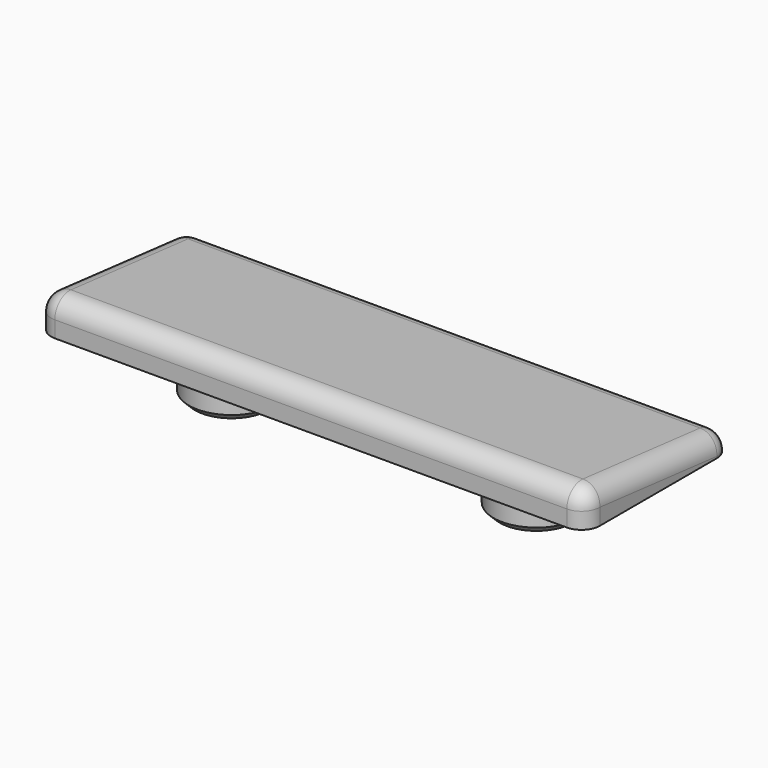
from build123d import *

# Parameters (mm, degrees)
F1_DEPTH     = 90
F3_R         = 7
F4_DEPTH     = 9
F5_R         = 3.35
F6_DEPTH     = 6
F7_SIZE      = 1
F8_R         = 3
F9_T1_DEPTH  = 84
F9_T3_DEPTH  = 24.1197014907
F9_T8_DEPTH  = 3
F9_T14_DEPTH = 3
F9_T20_DEPTH = 3
F9_T26_DEPTH = 3


# Not quite as in the source:
# - a fillet or chamfer that OpenCascade refuses, or shapes differently, is made with other operations: its cross-section is extruded or revolved along the edge and cut away or added


with BuildPart() as f1:
    # F0 (on Right) → F1 (new body)
    with BuildSketch(Plane.YZ):
        Polygon((-15, 6), (-15, 0), (15, 0), (15, 3), align=None)
    extrude(amount=F1_DEPTH)

    # F3 (on face) → F4 (join)
    with BuildSketch(Plane(origin=(0, 0, 0), x_dir=(1, 0, 0), z_dir=(0, 0, -1))):
        with Locations((70, 0)):
            Circle(F3_R)
        with Locations((20, 0)):
            Circle(F3_R)
    extrude(amount=F4_DEPTH)

    # F5 (on face) → F6 (cut)
    with BuildSketch(Plane(origin=(0, 0, -9), x_dir=(1, 0, 0), z_dir=(0, 0, -1))):
        with Locations((70, 0)):
            Circle(F5_R)
        with Locations((20, 0)):
            Circle(F5_R)
    extrude(amount=-F6_DEPTH, mode=Mode.SUBTRACT)

    # F7
    f7_edges = [f1.edges().sort_by_distance(p)[0] for p in [
        (63, 0, -9),
        (13, 0, -9),
    ]]
    chamfer(f7_edges, length=F7_SIZE)

    # F8
    f8_edges = [f1.edges().sort_by_distance(p)[0] for p in [
        (90, 15, 1.5),
        (0, 15, 1.5),
        (0, -15, 3),
        (90, -15, 3),
    ]]
    fillet(f8_edges, radius=F8_R)

    # F9: fillet of radius 3 on 4 edges, made by hand

    # F9_s2 → F9_t1 (cut)
    with BuildSketch(Plane.YZ.offset(3)):
        with BuildLine():
            ThreePointArc((15, 0.2850373137), (14.2243576007, 2.2980532759), (12.2985111571, 3.2701488843))
            Line((12.2985111571, 3.2701488843), (15, 3))
            Line((15, 3), (15, 0.2850373137))
        make_face()
        with BuildLine():
            ThreePointArc((-15, 2.6850373137), (-14.0130159623, 4.9093949143), (-11.7014888429, 5.6701488843))
            Line((-11.7014888429, 5.6701488843), (-15, 6))
            Line((-15, 6), (-15, 2.6850373137))
        make_face()
    extrude(amount=F9_T1_DEPTH, mode=Mode.SUBTRACT)

    # F9_s4 → F9_t3 (cut)
    with BuildSketch(Plane(origin=(0, 11.8529666026, -1.1852966603), x_dir=(1, 0, 0), z_dir=(0, -0.9950371902, 0.099503719))):
        with BuildLine():
            ThreePointArc((0, 1.4776673559), (0.8786796564, 3.5989876995), (3, 4.4776673559))
            Line((3, 4.4776673559), (0, 4.4776673559))
            Line((0, 4.4776673559), (0, 1.4776673559))
        make_face()
        with BuildLine():
            ThreePointArc((90, 1.4776673559), (89.1213203436, 3.5989876995), (87, 4.4776673559))
            Line((87, 4.4776673559), (90, 4.4776673559))
            Line((90, 4.4776673559), (90, 1.4776673559))
        make_face()
    extrude(amount=F9_T3_DEPTH, mode=Mode.SUBTRACT)


with BuildPart() as f9_tool6:
    # F9_s7 → F9_t8 (new body)
    with BuildSketch(Plane.YZ.offset(87)):
        Polygon((12, 0.2850373137), (15, 0.2850373137), (15, 3), (12.2985111571, 3.2701488843), align=None)
    extrude(amount=F9_T8_DEPTH)

    # F9_s9 → F9_t10 (revolve, cut)
    with BuildSketch(Plane(origin=(87, 12, 0.2850373137), x_dir=(0, -0.7414525336, -0.6710053208), z_dir=(0, -0.6710053208, 0.7414525336))):
        with BuildLine():
            ThreePointArc((0, -3), (3, 0), (0, 3))
            Line((0, 3), (0, -3))
        make_face()
    revolve(axis=Axis((87, 12, 0.2850373137), (1, 0, 0)), mode=Mode.SUBTRACT)


with BuildPart() as f1_1:
    add(f1.part)

    # F9_t5: cut F9_tool6
    add(f9_tool6.part, mode=Mode.SUBTRACT)


with BuildPart() as f9_tool12:
    # F9_s13 → F9_t14 (new body)
    with BuildSketch(Plane.YZ.offset(87)):
        Polygon((-12, 2.6850373137), (-15, 2.6850373137), (-15, 6), (-11.7014888429, 5.6701488843), align=None)
    extrude(amount=F9_T14_DEPTH)

    # F9_s15 → F9_t16 (revolve, cut)
    with BuildSketch(Plane(origin=(87, -12, 2.6850373137), x_dir=(0, 0.6710053208, -0.7414525336), z_dir=(0, -0.7414525336, -0.6710053208))):
        with BuildLine():
            ThreePointArc((0, -3), (3, 0), (0, 3))
            Line((0, 3), (0, -3))
        make_face()
    revolve(axis=Axis((87, -12, 2.6850373137), (1, 0, 0)), mode=Mode.SUBTRACT)


with BuildPart() as f1_2:
    add(f1_1.part)

    # F9_t11: cut F9_tool12
    add(f9_tool12.part, mode=Mode.SUBTRACT)


with BuildPart() as f9_tool18:
    # F9_s19 → F9_t20 (new body)
    with BuildSketch(Plane.YZ.offset(3)):
        Polygon((12, 0.2850373137), (15, 0.2850373137), (15, 3), (12.2985111571, 3.2701488843), align=None)
    extrude(amount=-F9_T20_DEPTH)

    # F9_s21 → F9_t22 (revolve, cut)
    with BuildSketch(Plane(origin=(3, 12, 0.2850373137), x_dir=(0, -0.7414525336, -0.6710053208), z_dir=(0, 0.6710053208, -0.7414525336))):
        with BuildLine():
            ThreePointArc((0, -3), (3, 0), (0, 3))
            Line((0, 3), (0, -3))
        make_face()
    revolve(axis=Axis((3, 12, 0.2850373137), (-1, 0, 0)), mode=Mode.SUBTRACT)


with BuildPart() as f1_3:
    add(f1_2.part)

    # F9_t17: cut F9_tool18
    add(f9_tool18.part, mode=Mode.SUBTRACT)


with BuildPart() as f9_tool24:
    # F9_s25 → F9_t26 (new body)
    with BuildSketch(Plane.YZ.offset(3)):
        Polygon((-12, 2.6850373137), (-15, 2.6850373137), (-15, 6), (-11.7014888429, 5.6701488843), align=None)
    extrude(amount=-F9_T26_DEPTH)

    # F9_s27 → F9_t28 (revolve, cut)
    with BuildSketch(Plane(origin=(3, -12, 2.6850373137), x_dir=(0, 0.6710053208, -0.7414525336), z_dir=(0, 0.7414525336, 0.6710053208))):
        with BuildLine():
            ThreePointArc((0, -3), (3, 0), (0, 3))
            Line((0, 3), (0, -3))
        make_face()
    revolve(axis=Axis((3, -12, 2.6850373137), (-1, 0, 0)), mode=Mode.SUBTRACT)


with BuildPart() as f1_4:
    add(f1_3.part)

    # F9_t23: cut F9_tool24
    add(f9_tool24.part, mode=Mode.SUBTRACT)


solid = f1_4.part
